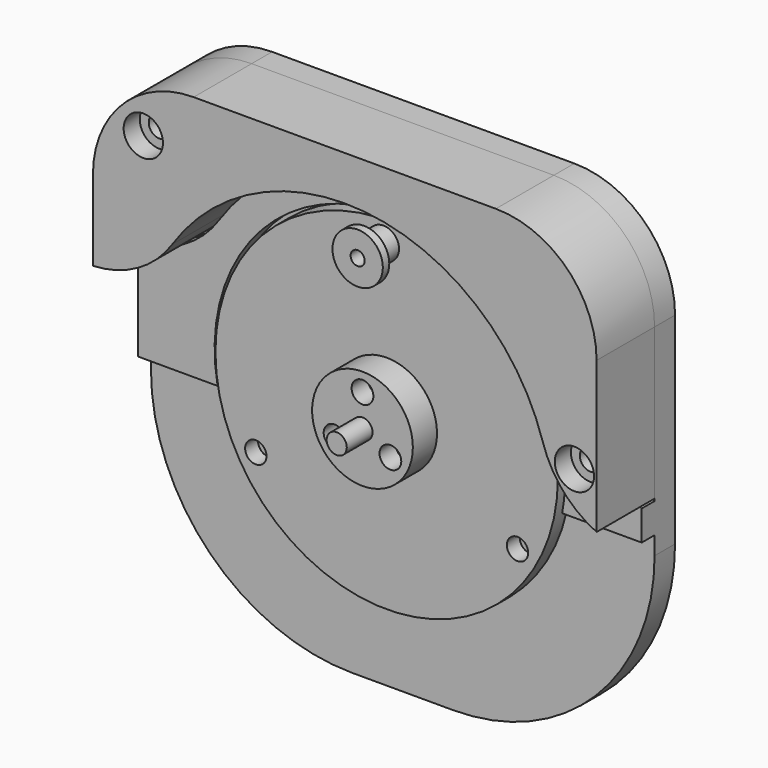
from build123d import *

# Parameters (mm, degrees)
F0_W              = 125
F0_H              = 125
F3_DEPTH          = 6.35
F4_D              = 3.4
F4_CBORE_D        = 6.5
F4_CBORE_DEPTH    = 3
F1_R              = 11.5
F5_DEPTH          = 6.351
F6_R              = 2.5
F7_DEPTH          = 20.5
F9_DEPTH          = 18
F11_R             = 42.5
F11_R_2           = 2.655
F11_R_3           = 2.5
F12_DEPTH         = 4
F13_R             = 12.5
F13_R_2           = 2.5
F14_DEPTH         = 7.5
F15_R             = 2.7
F16_DEPTH         = 5
F18_R             = 1.5
F19_DEPTH         = 13
F20_R             = 2.7
F20_R_2           = 1.5
F21_DEPTH         = 5
F23_D             = 5.3
F23_CBORE_D       = 9.75
F23_CBORE_DEPTH   = 5
F23_2_D           = 5.3
F23_2_CBORE_D     = 9.75
F23_2_CBORE_DEPTH = 5
F27_F1_R          = 25
F27_F2_R          = 25
F27_2_T1_DEPTH    = 88.3223792338
F27_2_T3_DEPTH    = 95.1320995715
F27_2_T5_DEPTH    = 143
F30_DEPTH         = 4
F31_R             = 50
F33_R             = 3.875
F33_R_2           = 1.75
F34_DEPTH         = 6
F35_R             = 6.25
F35_R_2           = 1.75
F36_DEPTH         = 2


# Not quite as in the source:
# - a fillet or chamfer that OpenCascade refuses, or shapes differently, is made with other operations: its cross-section is extruded or revolved along the edge and cut away or added


with BuildPart() as f3:
    # F0 (on Front) → F3 (new body)
    with BuildSketch(Plane.XZ):
        Rectangle(F0_W, F0_H)
    extrude(amount=-F3_DEPTH)

    # F4 (through all)
    with Locations(Plane.XZ):
        with Locations((-16, 16), (16, 16), (-16, -16), (16, -16)):
            CounterBoreHole(F4_D / 2, F4_CBORE_D / 2, F4_CBORE_DEPTH)

    # F1 (on Front) → F5 (cut, through all)
    with BuildSketch(Plane.XZ):
        Circle(F1_R)
    extrude(amount=-F5_DEPTH, mode=Mode.SUBTRACT)

    # F23 (through all)
    with Locations(Plane.XZ.offset(18)):
        with Locations((57, 12), (-50, 50)):
            CounterBoreHole(F23_D / 2, F23_CBORE_D / 2, F23_CBORE_DEPTH)

    # F27: fillet of radius 25 on 2 edges, made by hand

    # F27_f1
    f27_f1_edges = [f3.edges().sort_by_distance(p)[0] for p in [
        (62.5, 3.175, 62.5),
    ]]
    fillet(f27_f1_edges, radius=F27_F1_R)

    # F27_f2
    f27_f2_edges = [f3.edges().sort_by_distance(p)[0] for p in [
        (-62.5, 3.175, 62.5),
    ]]
    fillet(f27_f2_edges, radius=F27_F2_R)

    # F29 (on face) → F30 (join)
    with BuildSketch(Plane.XZ):
        with BuildLine():
            ThreePointArc((48.712, 15.1043389792), (7.3176199351, 50.4722937708), (-42.4167281702, 28.3164470111))
            ThreePointArc((-42.4167281702, 28.3164470111), (-51.1065410497, 20.2590031688), (-62.5, 16.9995028545))
            Line((-62.5, 16.9995028545), (-62.5, -8.0004971455))
            Line((-62.5, -8.0004971455), (-42.757947161, -8.0004971455))
            ThreePointArc((-42.757947161, -8.0004971455), (-4.0174182316, 43.3140895178), (43.5, 0))
            ThreePointArc((43.5, 0), (43.3140872238, -4.0174429644), (42.7579380243, -8.0005459758))
            Line((42.7579380243, -8.0005459758), (62.5, -8.0005459758))
            Line((62.5, -8.0005459758), (62.5, -0.5505459758))
            ThreePointArc((62.5, -0.5505459758), (53.9319006133, 5.8024377362), (48.712, 15.1043389792))
        make_face()
    extrude(amount=F30_DEPTH)

    # F31
    f31_edges = [f3.edges().sort_by_distance(p)[0] for p in [
        (-62.5, 3.175, -62.5),
        (62.5, 3.175, -62.5),
    ]]
    fillet(f31_edges, radius=F31_R)


with BuildPart() as f7:
    # F6 (on Front) → F7 (new body)
    with BuildSketch(Plane.XZ):
        Circle(F6_R)
    extrude(amount=F7_DEPTH)


with BuildPart() as f9:
    # F8 (on Front) → F9 (new body)
    with BuildSketch(Plane.XZ):
        with BuildLine():
            ThreePointArc((-48.4355241532, 17.5), (8.8831443225, 50.7280962283), (51.5, 0))
            Line((51.5, 0), (62.5, 0))
            Line((62.5, 0), (62.5, 62.5))
            Line((62.5, 62.5), (-62.5, 62.5))
            Line((-62.5, 62.5), (-62.5, 17.5))
            Line((-62.5, 17.5), (-48.4355241532, 17.5))
        make_face()
    extrude(amount=F9_DEPTH)

    # F23#2 (through all)
    with Locations(Plane.XZ.offset(18)):
        with Locations((57, 12), (-50, 50)):
            CounterBoreHole(F23_2_D / 2, F23_2_CBORE_D / 2, F23_2_CBORE_DEPTH)

    # F27#2: fillet of radius 25 on 4 edges, made by hand

    # F27_2_s2 → F27_2_t1 (cut)
    with BuildSketch(Plane.XZ.offset(-35.1611896169)):
        with BuildLine():
            ThreePointArc((-42.8325784464, 28.5940592367), (-51.3423848386, 20.7000270405), (-62.5, 17.5))
            Line((-62.5, 17.5), (-48.4355241532, 17.5))
            ThreePointArc((-48.4355241532, 17.5), (-45.9699486145, 23.2166712596), (-42.8325784464, 28.5940592367))
        make_face()
    extrude(amount=F27_2_T1_DEPTH, mode=Mode.SUBTRACT)

    # F27_2_s4 → F27_2_t3 (cut)
    with BuildSketch(Plane.XZ.offset(-38.5660497858)):
        with BuildLine():
            ThreePointArc((49.1895686275, 15.2524207339), (54.2319111507, 6.2186936243), (62.5, 0))
            Line((62.5, 0), (51.5, 0))
            ThreePointArc((51.5, 0), (50.9191161761, 7.7132099572), (49.1895686275, 15.2524207339))
        make_face()
    extrude(amount=F27_2_T3_DEPTH, mode=Mode.SUBTRACT)

    # F27_2_s6 → F27_2_t5 (cut)
    with BuildSketch(Plane.XZ.offset(-62.5)):
        with BuildLine():
            ThreePointArc((-62.5, 37.5), (-55.1776695297, 55.1776695297), (-37.5, 62.5))
            Line((-37.5, 62.5), (-62.5, 62.5))
            Line((-62.5, 62.5), (-62.5, 37.5))
        make_face()
        with BuildLine():
            ThreePointArc((62.5, 37.5), (55.1776695297, 55.1776695297), (37.5, 62.5))
            Line((37.5, 62.5), (62.5, 62.5))
            Line((62.5, 62.5), (62.5, 37.5))
        make_face()
    extrude(amount=F27_2_T5_DEPTH, mode=Mode.SUBTRACT)


with BuildPart() as f12:
    # F11 (on offset) → F12 (new body)
    with BuildSketch(Plane.XZ.offset(1)):
        Circle(F11_R)
        with Locations((-32.4759526419, -18.75)):
            Circle(F11_R_2, mode=Mode.SUBTRACT)
        with Locations((32.4759526419, -18.75)):
            Circle(F11_R_2, mode=Mode.SUBTRACT)
        Circle(F11_R_3, mode=Mode.SUBTRACT)
        with Locations((0, 37.8914289176)):
            Circle(F11_R_2, mode=Mode.SUBTRACT)
    extrude(amount=F12_DEPTH)

    # F13 (on face) → F14 (join)
    with BuildSketch(Plane.XZ.offset(5)):
        Circle(F13_R)
        Circle(F13_R_2, mode=Mode.SUBTRACT)
    extrude(amount=F14_DEPTH)

    # F15 (on face) → F16 (cut)
    with BuildSketch(Plane.XZ.offset(12.5)):
        with Locations((0, 8)):
            Circle(F15_R)
        with Locations((6.9282032303, -4)):
            Circle(F15_R)
        with Locations((-6.9282032303, -4)):
            Circle(F15_R)
    extrude(amount=-F16_DEPTH, mode=Mode.SUBTRACT)

    # F18 (on offset) → F19 (cut)
    with BuildSketch(Plane.XY.offset(-13)):
        with Locations((0, -8.75)):
            Circle(F18_R)
    extrude(amount=F19_DEPTH, mode=Mode.SUBTRACT)

    # F20 (on offset) → F21 (cut)
    with BuildSketch(Plane.XY.offset(-13)):
        with Locations((0, -8.75)):
            Circle(F20_R)
        with Locations((0, -8.75)):
            Circle(F20_R_2, mode=Mode.SUBTRACT)
        with Locations((0, -8.75)):
            Circle(F20_R_2)
    extrude(amount=F21_DEPTH, mode=Mode.SUBTRACT)


with BuildPart() as f34:
    # F33 (on offset) → F34 (new body)
    with BuildSketch(Plane.XZ.offset(6)):
        with Locations((0, 37.8914289176)):
            Circle(F33_R)
        with Locations((0, 37.8914289176)):
            Circle(F33_R_2, mode=Mode.SUBTRACT)
    extrude(amount=F34_DEPTH)

    # F35 (on face) → F36 (join)
    with BuildSketch(Plane.XZ.offset(12)):
        with Locations((0, 37.8914289176)):
            Circle(F35_R)
        with Locations((0, 37.8914289176)):
            Circle(F35_R_2, mode=Mode.SUBTRACT)
    extrude(amount=F36_DEPTH)


solid = Compound([f3.part, f7.part, f9.part, f12.part, f34.part])
